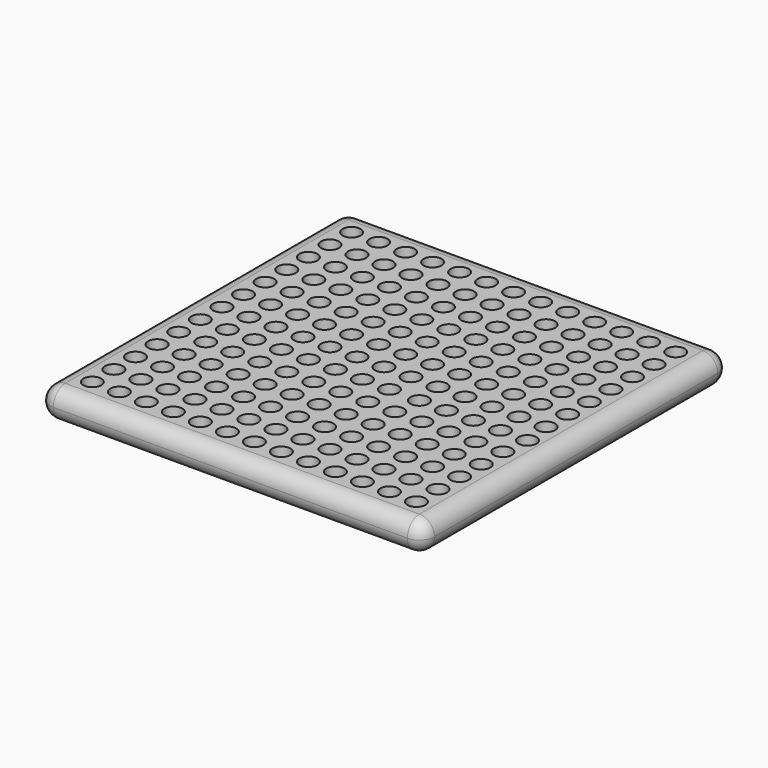
from build123d import *

# Parameters (mm, degrees)
F0_W     = 162.56
F0_H     = 162.56
F1_DEPTH = 12.7
F3_R     = 3.81
F4_DEPTH = 6.35
F5_R     = 6.34999


# Not quite as in the source:
# - a fillet or chamfer is up to 0.001 mm smaller than in the source, because OpenCascade refuses the exact size


with BuildPart() as f1:
    # F0 (on Top) → F1 (new body)
    with BuildSketch(Plane.XY):
        with Locations((-63.3368934822, 92.4975652182)):
            Rectangle(F0_W, F0_H)
    extrude(amount=F1_DEPTH)

    # F3 (on face) → F4 (cut)
    with BuildSketch(Plane.XY.offset(12.7)):
        with Locations((-131.9168934822, 23.9175652182)):
            Circle(F3_R)
        with Locations((-86.1968934822, 23.9175652182)):
            Circle(F3_R)
        with Locations((-40.4768934822, 23.9175652182)):
            Circle(F3_R)
        with Locations((5.2431065178, 23.9175652182)):
            Circle(F3_R)
        with Locations((-109.0568934822, 23.9175652182)):
            Circle(F3_R)
        with Locations((-63.3368934822, 23.9175652182)):
            Circle(F3_R)
        with Locations((-17.6168934822, 23.9175652182)):
            Circle(F3_R)
        with Locations((-131.9168934822, 46.7775652182)):
            Circle(F3_R)
        with Locations((-131.9168934822, 69.6375652182)):
            Circle(F3_R)
        with Locations((-131.9168934822, 92.4975652182)):
            Circle(F3_R)
        with Locations((-131.9168934822, 115.3575652182)):
            Circle(F3_R)
        with Locations((-131.9168934822, 138.2175652182)):
            Circle(F3_R)
        with Locations((-131.9168934822, 161.0775652182)):
            Circle(F3_R)
        with Locations((-109.0568934822, 46.7775652182)):
            Circle(F3_R)
        with Locations((-109.0568934822, 69.6375652182)):
            Circle(F3_R)
        with Locations((-109.0568934822, 92.4975652182)):
            Circle(F3_R)
        with Locations((-109.0568934822, 115.3575652182)):
            Circle(F3_R)
        with Locations((-109.0568934822, 138.2175652182)):
            Circle(F3_R)
        with Locations((-109.0568934822, 161.0775652182)):
            Circle(F3_R)
        with Locations((-86.1968934822, 46.7775652182)):
            Circle(F3_R)
        with Locations((-63.3368934822, 46.7775652182)):
            Circle(F3_R)
        with Locations((-40.4768934822, 46.7775652182)):
            Circle(F3_R)
        with Locations((188.1231065178, 46.7775652182)):
            Circle(F3_R)
        with Locations((5.2431065178, 46.7775652182)):
            Circle(F3_R)
        with Locations((-17.6168934822, 46.7775652182)):
            Circle(F3_R)
        with Locations((-86.1968934822, 161.0775652182)):
            Circle(F3_R)
        with Locations((-86.1968934822, 138.2175652182)):
            Circle(F3_R)
        with Locations((-86.1968934822, 115.3575652182)):
            Circle(F3_R)
        with Locations((-86.1968934822, 92.4975652182)):
            Circle(F3_R)
        with Locations((-86.1968934822, 69.6375652182)):
            Circle(F3_R)
        with Locations((-63.3368934822, 69.6375652182)):
            Circle(F3_R)
        with Locations((-40.4768934822, 69.6375652182)):
            Circle(F3_R)
        with Locations((-17.6168934822, 69.6375652182)):
            Circle(F3_R)
        with Locations((5.2431065178, 69.6375652182)):
            Circle(F3_R)
        with Locations((-63.3368934822, 92.4975652182)):
            Circle(F3_R)
        with Locations((-40.4768934822, 92.4975652182)):
            Circle(F3_R)
        with Locations((-17.6168934822, 92.4975652182)):
            Circle(F3_R)
        with Locations((5.2431065178, 92.4975652182)):
            Circle(F3_R)
        with Locations((-17.6168934822, 161.0775652182)):
            Circle(F3_R)
        with Locations((-63.3368934822, 115.3575652182)):
            Circle(F3_R)
        with Locations((-63.3368934822, 161.0775652182)):
            Circle(F3_R)
        with Locations((-17.6168934822, 138.2175652182)):
            Circle(F3_R)
        with Locations((-40.4768934822, 138.2175652182)):
            Circle(F3_R)
        with Locations((-40.4768934822, 161.0775652182)):
            Circle(F3_R)
        with Locations((5.2431065178, 115.3575652182)):
            Circle(F3_R)
        with Locations((5.2431065178, 138.2175652182)):
            Circle(F3_R)
        with Locations((-40.4768934822, 115.3575652182)):
            Circle(F3_R)
        with Locations((-63.3368934822, 138.2175652182)):
            Circle(F3_R)
        with Locations((5.2431065178, 161.0775652182)):
            Circle(F3_R)
        with Locations((-17.6168934822, 115.3575652182)):
            Circle(F3_R)
        with Locations((-120.4868934822, 161.0775652182)):
            Circle(F3_R)
        with Locations((-131.9168934822, 149.6475652182)):
            Circle(F3_R)
        with Locations((-120.4868934822, 149.6475652182)):
            Circle(F3_R)
        with Locations((-109.0568934822, 149.6475652182)):
            Circle(F3_R)
        with Locations((-120.4868934822, 138.2175652182)):
            Circle(F3_R)
        with Locations((-97.6268934822, 161.0775652182)):
            Circle(F3_R)
        with Locations((-97.6268934822, 149.6475652182)):
            Circle(F3_R)
        with Locations((-97.6268934822, 138.2175652182)):
            Circle(F3_R)
        with Locations((-86.1968934822, 149.6475652182)):
            Circle(F3_R)
        with Locations((-74.7668934822, 161.0775652182)):
            Circle(F3_R)
        with Locations((-74.7668934822, 149.6475652182)):
            Circle(F3_R)
        with Locations((-74.7668934822, 138.2175652182)):
            Circle(F3_R)
        with Locations((-63.3368934822, 149.6475652182)):
            Circle(F3_R)
        with Locations((-51.9068934822, 161.0775652182)):
            Circle(F3_R)
        with Locations((-51.9068934822, 149.6475652182)):
            Circle(F3_R)
        with Locations((-51.9068934822, 138.2175652182)):
            Circle(F3_R)
        with Locations((-40.4768934822, 149.6475652182)):
            Circle(F3_R)
        with Locations((-29.0468934822, 161.0775652182)):
            Circle(F3_R)
        with Locations((-29.0468934822, 149.6475652182)):
            Circle(F3_R)
        with Locations((-29.0468934822, 138.2175652182)):
            Circle(F3_R)
        with Locations((-17.6168934822, 149.6475652182)):
            Circle(F3_R)
        with Locations((-6.1868934822, 161.0775652182)):
            Circle(F3_R)
        with Locations((-6.1868934822, 149.6475652182)):
            Circle(F3_R)
        with Locations((5.2431065178, 149.6475652182)):
            Circle(F3_R)
        with Locations((-6.1868934822, 138.2175652182)):
            Circle(F3_R)
        with Locations((-131.9168934822, 126.7875652182)):
            Circle(F3_R)
        with Locations((-131.9168934822, 103.9275652182)):
            Circle(F3_R)
        with Locations((-120.4868934822, 126.7875652182)):
            Circle(F3_R)
        with Locations((-109.0568934822, 126.7875652182)):
            Circle(F3_R)
        with Locations((-120.4868934822, 115.3575652182)):
            Circle(F3_R)
        with Locations((-120.4868934822, 103.9275652182)):
            Circle(F3_R)
        with Locations((-109.0568934822, 103.9275652182)):
            Circle(F3_R)
        with Locations((-120.4868934822, 92.4975652182)):
            Circle(F3_R)
        with Locations((-120.4868934822, 81.0675652182)):
            Circle(F3_R)
        with Locations((-109.0568934822, 81.0675652182)):
            Circle(F3_R)
        with Locations((-131.9168934822, 81.0675652182)):
            Circle(F3_R)
        with Locations((-120.4868934822, 69.6375652182)):
            Circle(F3_R)
        with Locations((-109.0568934822, 58.2075652182)):
            Circle(F3_R)
        with Locations((-120.4868934822, 58.2075652182)):
            Circle(F3_R)
        with Locations((-131.9168934822, 58.2075652182)):
            Circle(F3_R)
        with Locations((-120.4868934822, 46.7775652182)):
            Circle(F3_R)
        with Locations((-120.4868934822, 23.9175652182)):
            Circle(F3_R)
        with Locations((-120.4868934822, 35.3475652182)):
            Circle(F3_R)
        with Locations((-109.0568934822, 35.3475652182)):
            Circle(F3_R)
        with Locations((-131.9168934822, 35.3475652182)):
            Circle(F3_R)
        with Locations((-97.6268934822, 126.7875652182)):
            Circle(F3_R)
        with Locations((-86.1968934822, 126.7875652182)):
            Circle(F3_R)
        with Locations((-97.6268934822, 115.3575652182)):
            Circle(F3_R)
        with Locations((-74.7668934822, 115.3575652182)):
            Circle(F3_R)
        with Locations((-74.7668934822, 126.7875652182)):
            Circle(F3_R)
        with Locations((-63.3368934822, 126.7875652182)):
            Circle(F3_R)
        with Locations((-51.9068934822, 126.7875652182)):
            Circle(F3_R)
        with Locations((-51.9068934822, 115.3575652182)):
            Circle(F3_R)
        with Locations((-40.4768934822, 126.7875652182)):
            Circle(F3_R)
        with Locations((-29.0468934822, 126.7875652182)):
            Circle(F3_R)
        with Locations((-17.6168934822, 126.7875652182)):
            Circle(F3_R)
        with Locations((-29.0468934822, 115.3575652182)):
            Circle(F3_R)
        with Locations((-6.1868934822, 126.7875652182)):
            Circle(F3_R)
        with Locations((5.2431065178, 126.7875652182)):
            Circle(F3_R)
        with Locations((-6.1868934822, 115.3575652182)):
            Circle(F3_R)
        with Locations((-97.6268934822, 103.9275652182)):
            Circle(F3_R)
        with Locations((-97.6268934822, 92.4975652182)):
            Circle(F3_R)
        with Locations((-86.1968934822, 103.9275652182)):
            Circle(F3_R)
        with Locations((-74.7668934822, 103.9275652182)):
            Circle(F3_R)
        with Locations((-74.7668934822, 92.4975652182)):
            Circle(F3_R)
        with Locations((-63.3368934822, 103.9275652182)):
            Circle(F3_R)
        with Locations((-51.9068934822, 103.9275652182)):
            Circle(F3_R)
        with Locations((-51.9068934822, 92.4975652182)):
            Circle(F3_R)
        with Locations((-40.4768934822, 103.9275652182)):
            Circle(F3_R)
        with Locations((-29.0468934822, 103.9275652182)):
            Circle(F3_R)
        with Locations((-29.0468934822, 92.4975652182)):
            Circle(F3_R)
        with Locations((-17.6168934822, 103.9275652182)):
            Circle(F3_R)
        with Locations((-6.1868934822, 103.9275652182)):
            Circle(F3_R)
        with Locations((5.2431065178, 103.9275652182)):
            Circle(F3_R)
        with Locations((-6.1868934822, 92.4975652182)):
            Circle(F3_R)
        with Locations((-39.2068934822, 81.0675652182)):
            Circle(F3_R)
        with Locations((-27.7768934822, 81.0675652182)):
            Circle(F3_R)
        with Locations((-29.0468934822, 69.6375652182)):
            Circle(F3_R)
        with Locations((-16.3468934822, 81.0675652182)):
            Circle(F3_R)
        with Locations((-4.9168934822, 81.0675652182)):
            Circle(F3_R)
        with Locations((6.5131065178, 81.0675652182)):
            Circle(F3_R)
        with Locations((-6.1868934822, 69.6375652182)):
            Circle(F3_R)
        with Locations((5.2431065178, 58.2075652182)):
            Circle(F3_R)
        with Locations((-6.1868934822, 58.2075652182)):
            Circle(F3_R)
        with Locations((-29.0468934822, 58.2075652182)):
            Circle(F3_R)
        with Locations((-17.6168934822, 58.2075652182)):
            Circle(F3_R)
        with Locations((-29.0468934822, 46.7775652182)):
            Circle(F3_R)
        with Locations((-6.1868934822, 46.7775652182)):
            Circle(F3_R)
        with Locations((-29.0468934822, 35.3475652182)):
            Circle(F3_R)
        with Locations((-40.4768934822, 35.3475652182)):
            Circle(F3_R)
        with Locations((-17.6168934822, 35.3475652182)):
            Circle(F3_R)
        with Locations((-6.1868934822, 35.3475652182)):
            Circle(F3_R)
        with Locations((5.2431065178, 35.3475652182)):
            Circle(F3_R)
        with Locations((-29.0468934822, 23.9175652182)):
            Circle(F3_R)
        with Locations((-6.1868934822, 23.9175652182)):
            Circle(F3_R)
        with Locations((-40.4768934822, 58.2075652182)):
            Circle(F3_R)
        with Locations((-86.1968934822, 81.0675652182)):
            Circle(F3_R)
        with Locations((-74.7668934822, 81.0675652182)):
            Circle(F3_R)
        with Locations((-63.3368934822, 81.0675652182)):
            Circle(F3_R)
        with Locations((-97.6268934822, 81.0675652182)):
            Circle(F3_R)
        with Locations((-97.6268934822, 69.6375652182)):
            Circle(F3_R)
        with Locations((-74.7668934822, 69.6375652182)):
            Circle(F3_R)
        with Locations((-51.9068934822, 69.6375652182)):
            Circle(F3_R)
        with Locations((-51.9068934822, 81.0675652182)):
            Circle(F3_R)
        with Locations((-97.6268934822, 58.2075652182)):
            Circle(F3_R)
        with Locations((-86.1968934822, 58.2075652182)):
            Circle(F3_R)
        with Locations((-74.7668934822, 58.2075652182)):
            Circle(F3_R)
        with Locations((-63.3368934822, 58.2075652182)):
            Circle(F3_R)
        with Locations((-51.9068934822, 58.2075652182)):
            Circle(F3_R)
        with Locations((-51.9068934822, 46.7775652182)):
            Circle(F3_R)
        with Locations((-51.9068934822, 35.3475652182)):
            Circle(F3_R)
        with Locations((-51.9068934822, 23.9175652182)):
            Circle(F3_R)
        with Locations((-63.3368934822, 35.3475652182)):
            Circle(F3_R)
        with Locations((-74.7668934822, 46.7775652182)):
            Circle(F3_R)
        with Locations((-74.7668934822, 35.3475652182)):
            Circle(F3_R)
        with Locations((-74.7668934822, 23.9175652182)):
            Circle(F3_R)
        with Locations((-86.1968934822, 35.3475652182)):
            Circle(F3_R)
        with Locations((-97.6268934822, 46.7775652182)):
            Circle(F3_R)
        with Locations((-97.6268934822, 35.3475652182)):
            Circle(F3_R)
        with Locations((-97.6268934822, 23.9175652182)):
            Circle(F3_R)
    extrude(amount=-F4_DEPTH, mode=Mode.SUBTRACT)

    # F5 (radius 6.35 in the source; OpenCascade refuses exactly that, so slightly less here)
    f5_edges = [f1.edges().sort_by_distance(p)[0] for p in [
        (-144.616893, 11.217565, 6.35),
        (17.943107, 11.217565, 6.35),
        (-63.336893, 11.217565, 0),
        (-63.336893, 11.217565, 12.7),
        (-144.616893, 173.777565, 6.35),
        (-144.616893, 92.497565, 0),
        (-144.616893, 92.497565, 12.7),
        (17.943107, 173.777565, 6.35),
        (-63.336893, 173.777565, 0),
        (-63.336893, 173.777565, 12.7),
        (17.943107, 92.497565, 0),
        (17.943107, 92.497565, 12.7),
    ]]
    fillet(f5_edges, radius=F5_R)


solid = f1.part
